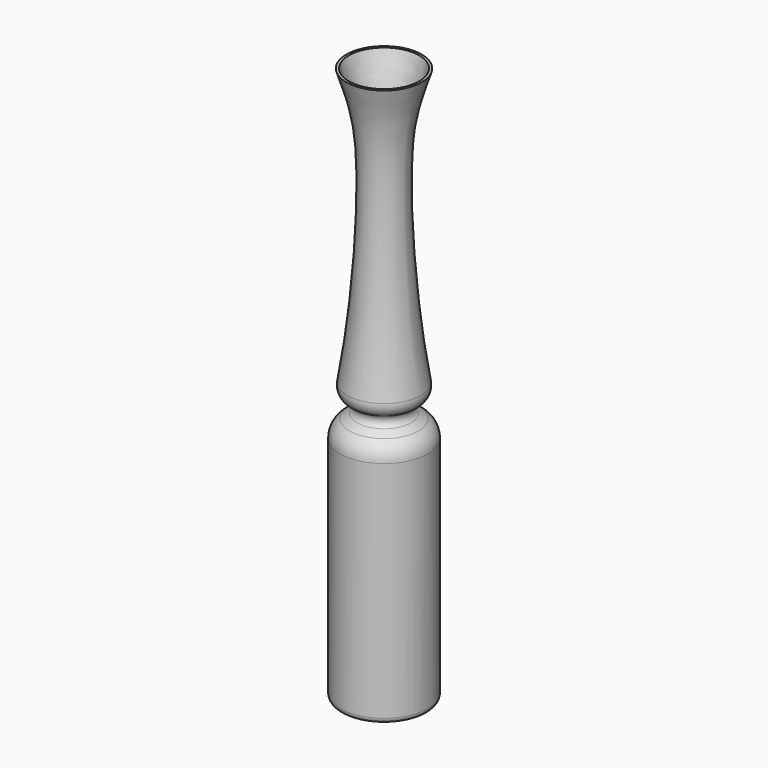
from build123d import *


# Not quite as in the source:
# - ends of sketch curves that miss each other by under 0.0002 mm in the source are joined
# - the dataset's text gives a spline's control points without its knots; the knots are read off the source's solid


with BuildPart() as f1:
    # F0 (on Front) → F1 (revolve)
    with BuildSketch(Plane.XZ):
        with BuildLine():
            ThreePointArc((5.3665031115, 0.0459550024), (6.0543176759, 0.1350314372), (6.375, 0.75))
            Line((6.375, 0.75), (6.375, 33.5))
            ThreePointArc((6.375, 33.5), (6.0150603981, 34.9248091431), (5.0216126038, 36.0077214624))
            Line((5.0216126038, 36.0077214624), (3.9511291321, 36.7106191339))
            ThreePointArc((3.9511291321, 36.7106191339), (3.5050589675, 37.646986936), (4.129309804, 38.4752828647))
            ThreePointArc((4.129309804, 38.4752828647), (5.135512873, 39.3601953563), (5.3572629788, 40.6816875524))
            add(Edge.make_bspline(
                [(5.3572629788, 40.6816875524), (3.5919283633, 50.646196206), (2.3467552195, 71.9217737234), (4.3341060529, 77.2873032352), (5.5, 81)],
                knots=[0.0165250757, 0.0165250757, 0.0165250757, 0.0165250757, 0.638652351, 1, 1, 1, 1], degree=3))
            Line((5.5, 81), (5.1331190125, 81))
            add(Edge.make_bspline(
                [(5.0038158008, 40.6704484598), (4.6984079165, 42.3994911801), (4.1015811021, 46.3621189154), (3.4065256445, 52.8331604138), (2.9434400764, 59.5709572319), (2.7919372258, 64.7457686722), (2.8192744411, 68.3836267885), (2.9000021009, 70.4005298819), (3.0040929662, 71.8283670538), (3.1347752343, 73.1381118153), (3.4334170243, 75.1798025444), (4.0529129834, 77.6404662934), (4.7441946947, 79.7636672453), (5.1331190125, 81)],
                knots=[0.0175574673, 0.0175574673, 0.0175574673, 0.0175574673, 0.125, 0.25, 0.375, 0.5, 0.5625, 0.625, 0.65625, 0.6875, 0.75, 0.875, 0.996577621, 0.996577621, 0.996577621, 0.996577621], degree=3))
            ThreePointArc((5.0038158008, 40.6704484598), (4.8201347615, 39.74598328), (4.0600591191, 39.1886139901))
            ThreePointArc((4.0600591191, 39.1886139901), (2.8000187772, 37.554516415), (4.0446428571, 35.9086466))
            ThreePointArc((4.0446428571, 35.9086466), (5.3654907866, 35.0125959238), (5.875, 33.5))
            Line((5.875, 33.5), (5.875, 1.0658816932))
            ThreePointArc((5.875, 1.0658816932), (5.5849031426, 0.4984493944), (4.9550588179, 0.4013323147))
            ThreePointArc((4.9550588179, 0.4013323147), (2.5095058259, 0.9990528325), (0, 1.2))
            Line((0, 1.2), (0, 1))
            ThreePointArc((0, 1), (2.7253237195, 0.759633422), (5.3665031115, 0.0459550024))
        make_face()
    revolve(axis=Axis((0, 0, 41.3556105854), (0, 0, 1)))


solid = f1.part
